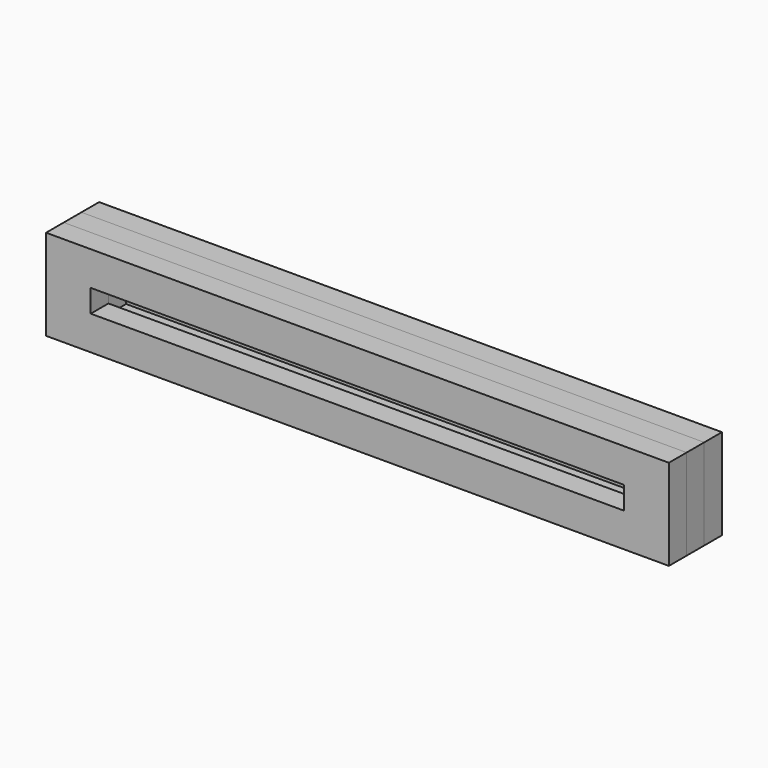
from build123d import *

# Parameters (mm, degrees)
F0_W     = 82.3
F0_H     = 12
F1_DEPTH = 2.92
F2_W     = 82.3
F2_H     = 12
F2_W_2   = 70.5
F2_H_2   = 5.5
F3_DEPTH = 2.92
F4_W     = 82.3
F4_H     = 12
F4_W_2   = 70.5
F4_H_2   = 1.25
F5_DEPTH = 2.92


# Not quite as in the source:
# - a feature names something its author has since deleted; it is built from what else it names


with BuildPart() as f1:
    # F0 (on Front) → F1 (new body)
    with BuildSketch(Plane.XZ):
        Rectangle(F0_W, F0_H)
    extrude(amount=F1_DEPTH)


with BuildPart() as f3:
    # F2 (on face) → F3 (new body)
    with BuildSketch(Plane.XZ.offset(2.92)):
        Rectangle(F2_W, F2_H)
        Rectangle(F2_W_2, F2_H_2, mode=Mode.SUBTRACT)
    extrude(amount=F3_DEPTH)


with BuildPart() as f5:
    # F4 (on face) → F5 (new body)
    with BuildSketch(Plane.XZ.offset(5.84)):
        Rectangle(F4_W, F4_H)
        Polygon((35.25, 1.5), (35.25, -1.5), (35.25, -2.75), (-35.25, -2.75), (-35.25, -1.5), (-35.25, 1.5), (-35.25, 2.75), (35.25, 2.75), align=None, mode=Mode.SUBTRACT)
        with Locations((0, 2.125)):
            Rectangle(F4_W_2, F4_H_2)
        with Locations((0, -2.125)):
            Rectangle(F4_W_2, F4_H_2)
    extrude(amount=F5_DEPTH)


solid = Compound([f1.part, f3.part, f5.part])
